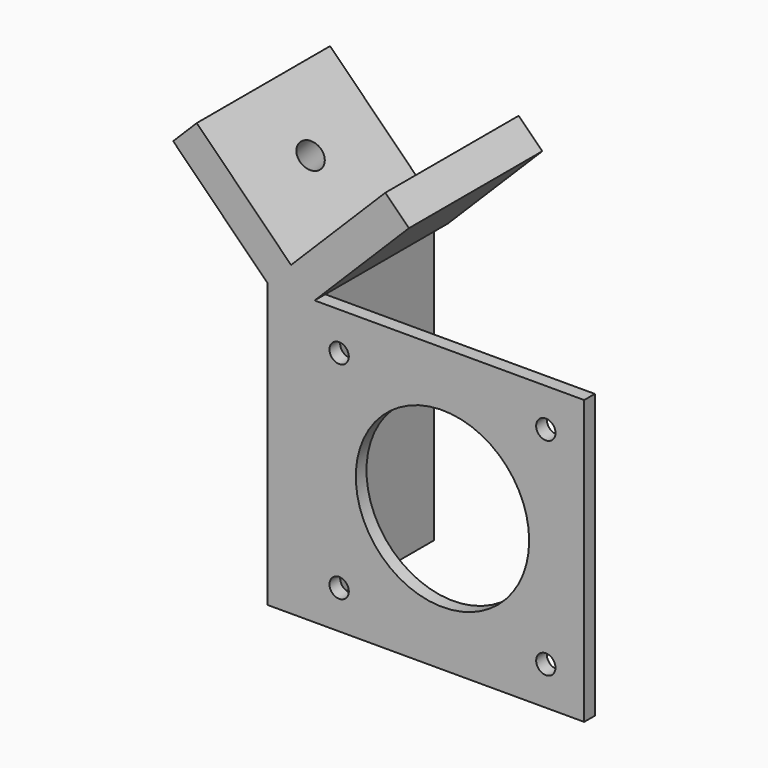
from build123d import *

# Parameters (mm, degrees)
F0_W     = 5
F0_H     = 42.5
F1_DEPTH = 25
F0_R     = 1.45
F0_R_2   = 13
F2_DEPTH = 2
F3_R     = 2
F4_DEPTH = 25


# Not quite as in the source:
# - a feature names something its author has since deleted; it is built from what else it names


with BuildPart() as f1:
    # F0 (on Front) → F1 (new body)
    with BuildSketch(Plane.XZ):
        Polygon((-51.006380532, 4.9005637974), (-36.8642449083, -9.2415718264), (-31.8642449083, -9.2415718264), (-29.7931770964, -9.2415718264), (-33.3287110023, -5.7060379204), (-47.4708466261, 8.4360977033), align=None)
        with Locations((-34.3642449083, -30.4915718264)):
            Rectangle(F0_W, F0_H)
        Polygon((-33.3287110023, -5.7060379204), (-29.7931770964, -9.2415718264), (-15.6510414727, 4.9005637974), (-19.1865753786, 8.4360977033), align=None)
    extrude(amount=-F1_DEPTH)

    # F0 (on Front) → F2 (join)
    with BuildSketch(Plane.XZ):
        Polygon((-29.7931770964, -9.2415718264), (-31.8642449083, -9.2415718264), (-31.8642449083, -51.7415718264), (10.6357550917, -51.7415718264), (10.6357550917, -9.2415718264), align=None)
        with Locations((-26.1142449083, -45.9915718264)):
            Circle(F0_R, mode=Mode.SUBTRACT)
        with Locations((4.8857550917, -45.9915718264)):
            Circle(F0_R, mode=Mode.SUBTRACT)
        with Locations((-10.6142449083, -30.4915718264)):
            Circle(F0_R_2, mode=Mode.SUBTRACT)
        with Locations((-26.1142449083, -14.9915718264)):
            Circle(F0_R, mode=Mode.SUBTRACT)
        with Locations((4.8857550917, -14.9915718264)):
            Circle(F0_R, mode=Mode.SUBTRACT)
    extrude(amount=-F2_DEPTH)

    # F3 (on face) → F4 (cut)
    with BuildSketch(Plane(origin=(-19.5173744614, 0, -19.5173744614), x_dir=(0.7071067812, 0, -0.7071067812), z_dir=(0.7071067812, 0, 0.7071067812))):
        with Locations((-29.5321794507, 12.5)):
            Circle(F3_R)
    extrude(amount=-F4_DEPTH, mode=Mode.SUBTRACT)


solid = f1.part
